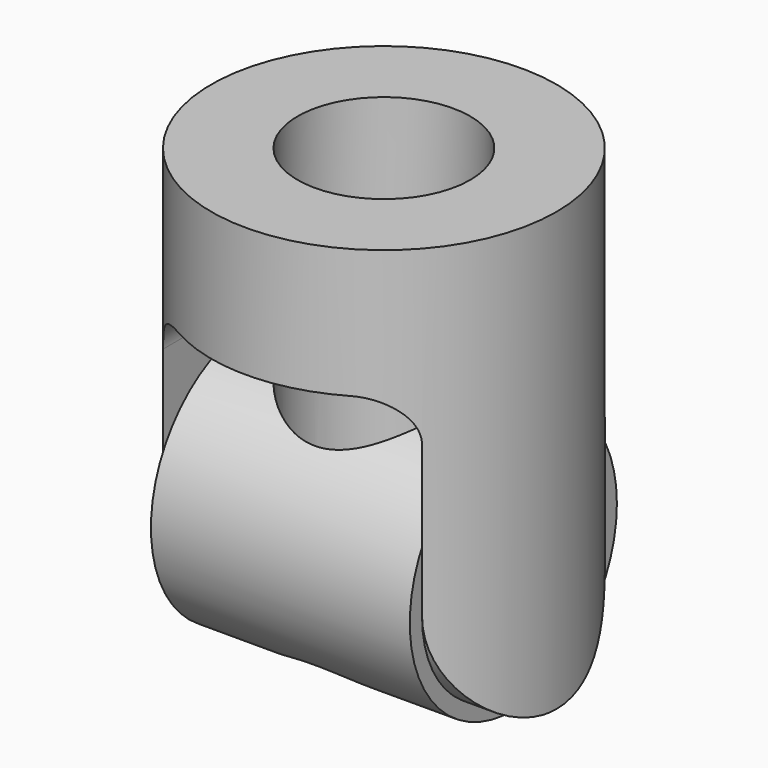
from build123d import *

# Parameters (mm, degrees)
F8_R           = 40
F9_DEPTH       = 60
F0_R           = 60
F0_R_2         = 9
F0_R_3         = 5
F1_DEPTH       = 60
F10_DEPTH      = 45
F8_R_2         = 80
F3_DEPTH       = 150
F3_DEPTH_BACK  = 60
F4_W           = 105.8300524426
F4_H           = 30
F11_DEPTH      = 25
F11_DEPTH_BACK = 145
F6_W           = 120
F6_H           = 150
F7_DEPTH       = 105.8300524426
F12_R          = 19.99999


# Not quite as in the source:
# - a fillet or chamfer is up to 0.001 mm smaller than in the source, because OpenCascade refuses the exact size


with BuildPart() as f9:
    # F8 (on Top) → F9 (new body, symmetric)
    with BuildSketch(Plane.XY):
        Circle(F8_R)
    extrude(amount=F9_DEPTH, both=True)


with BuildPart() as f1:
    # F0 (on Right) → F1 (new body, symmetric)
    with BuildSketch(Plane.YZ):
        Circle(F0_R)
        Circle(F0_R_2, mode=Mode.SUBTRACT)
        Circle(F0_R_2)
        Circle(F0_R_3, mode=Mode.SUBTRACT)
    extrude(amount=F1_DEPTH, both=True)

    # F2: cut F9
    add(f9.part, mode=Mode.SUBTRACT)

    # F0 (on Right) → F10 (cut, symmetric)
    with BuildSketch(Plane.YZ):
        Circle(F0_R_2)
        Circle(F0_R_3, mode=Mode.SUBTRACT)
    extrude(amount=F10_DEPTH, both=True, mode=Mode.SUBTRACT)


with BuildPart() as f3:
    # F8 (on Top) → F3 (new body, two sides)
    with BuildSketch(Plane.XY) as f3_sk:
        Circle(F8_R_2)
        Circle(F8_R, mode=Mode.SUBTRACT)
    extrude(amount=F3_DEPTH)
    extrude(f3_sk.sketch, amount=-F3_DEPTH_BACK)


with BuildPart() as f11:
    # F4 (on face) → F11 (new body, two sides)
    with BuildSketch(Plane.YZ.offset(60)) as f11_sk:
        with BuildLine():
            Line((-52.9150262213, 0), (52.9150262213, 0))
            ThreePointArc((52.9150262213, 0), (0, 52.9150262213), (-52.9150262213, 0))
        make_face()
        with BuildLine():
            ThreePointArc((-52.9150262213, 0), (0, -52.9150262213), (52.9150262213, 0))
            Line((52.9150262213, 0), (-52.9150262213, 0))
        make_face()
        with BuildLine():
            ThreePointArc((-52.9150262213, 0), (0, 52.9150262213), (52.9150262213, 0))
            Line((52.9150262213, 0), (52.9150262213, 90))
            Line((52.9150262213, 90), (-52.9150262213, 90))
            Line((-52.9150262213, 90), (-52.9150262213, 0))
        make_face()
        with Locations((0, 105)):
            Rectangle(F4_W, F4_H)
        Polygon((52.9150262213, 120), (52.9150262213, 90), (90, 90), (90, 150), (-90, 150), (-90, 90), (-52.9150262213, 90), (-52.9150262213, 120), align=None)
    extrude(amount=F11_DEPTH)
    extrude(f11_sk.sketch, amount=-F11_DEPTH_BACK)


with BuildPart() as f3_1:
    add(f3.part)

    # F5: intersect F11
    add(f11.part, mode=Mode.INTERSECT)

    # F6 (on face) → F7 (cut, through all)
    with BuildSketch(Plane.XZ.offset(52.9150262213)):
        with Locations((0, 15)):
            Rectangle(F6_W, F6_H)
    extrude(amount=-F7_DEPTH, mode=Mode.SUBTRACT)

    # F12 (radius 20 in the source; OpenCascade refuses exactly that, so slightly less here)
    f12_edges = [f3_1.edges().sort_by_distance(p)[0] for p in [
        (-60, 0, 90),
        (60, 0, 90),
    ]]
    fillet(f12_edges, radius=F12_R)


solid = Compound([f1.part, f3_1.part])
